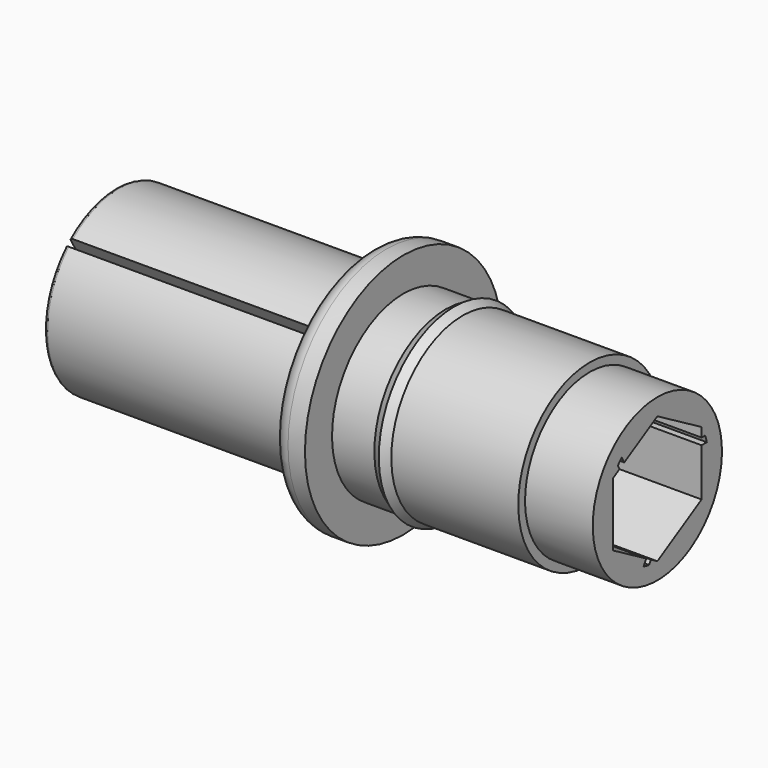
from build123d import *

# Parameters (mm, degrees)
F2_R     = 1
F4_DEPTH = 32
F5_DEPTH = 32
F6_DEPTH = 15
F7_DEPTH = 15
F8_DEPTH = 15
F9_R     = 0.2


with BuildPart() as f1:
    # F0 (on Front) → F1 (revolve)
    with BuildSketch(Plane.XZ):
        Polygon((-9.0454753935, 5.269), (-9.0454753935, 3.769), (22.9545246065, 3.769), (22.9545246065, 4.769), (18.9545246065, 4.769), (18.9545246065, 5.269), (11.4545246065, 5.269), (10.9545246065, 5.569), (10.4545246065, 5.269), (7.9545246065, 5.269), (7.9545246065, 7.269), (5.9545246065, 7.269), (5.9545246065, 5.269), align=None)
    revolve(axis=Axis((2.1683473801, 0, 0), (1, 0, 0)))

    # F2
    f2_edges = [f1.edges().sort_by_distance(p)[0] for p in [
        (5.954525, 0, -7.269),
    ]]
    fillet(f2_edges, radius=F2_R)

    # F3 (on face) → F4 (join)
    with BuildSketch(Plane(origin=(-9.0454753935, 0, 0), x_dir=(0, -1, 0), z_dir=(-1, 0, 0))):
        with BuildLine():
            ThreePointArc((3.769, 0), (3.6405744393, 0.975488981), (3.2640497469, 1.8845))
            Line((3.2640497469, 1.8845), (3.2640497469, -1.8845))
            ThreePointArc((3.2640497469, -1.8845), (3.6405744393, -0.975488981), (3.769, 0))
        make_face()
    extrude(amount=-F4_DEPTH)

    # F3 (on face) → F5 (join)
    with BuildSketch(Plane(origin=(-9.0454753935, 0, 0), x_dir=(0, -1, 0), z_dir=(-1, 0, 0))):
        with BuildLine():
            ThreePointArc((3.769, 0), (3.6405744393, 0.975488981), (3.2640497469, 1.8845))
            Line((3.2640497469, 1.8845), (3.2640497469, -1.8845))
            ThreePointArc((3.2640497469, -1.8845), (3.6405744393, -0.975488981), (3.769, 0))
        make_face()
        with BuildLine():
            Line((2.7877357748, 2.1595), (3.2640497469, 1.8845))
            ThreePointArc((3.2640497469, 1.8845), (3.1012168176, 2.1419185909), (2.9181290377, 2.3853477564))
            Line((2.9181290377, 2.3853477564), (2.7877357748, 2.1595))
        make_face()
        with BuildLine():
            ThreePointArc((1.0163546733, -3.6293779327), (2.3111934688, -2.9772043514), (3.2640497469, -1.8845))
            Line((3.2640497469, -1.8845), (0.8227241336, -3.294))
            Line((0.8227241336, -3.294), (1.0163546733, -3.6293779327))
        make_face()
        with BuildLine():
            Line((0, 3.769), (2.4413256133, 2.3595))
            Line((2.4413256133, 2.3595), (2.634956153, 2.6948779327))
            ThreePointArc((2.634956153, 2.6948779327), (1.4227378662, 3.4901544327), (0, 3.769))
        make_face()
        with BuildLine():
            Line((0.606707235, -3.7198477564), (0.4763139721, -3.494))
            Line((0.4763139721, -3.494), (0, -3.769))
            ThreePointArc((0, -3.769), (0.3043475037, -3.7566918422), (0.606707235, -3.7198477564))
        make_face()
        with BuildLine():
            Line((-3.2640497469, 1.8845), (0, 3.769))
            ThreePointArc((0, 3.769), (-1.8845, 3.2640497469), (-3.2640497469, 1.8845))
        make_face()
        with BuildLine():
            ThreePointArc((-3.2640497469, -1.8845), (-1.8845, -3.2640497469), (0, -3.769))
            Line((0, -3.769), (-3.2640497469, -1.8845))
        make_face()
        with BuildLine():
            Line((-3.2640497469, 1.3345), (-3.2640497469, 1.8845))
            ThreePointArc((-3.2640497469, 1.8845), (-3.4055643214, 1.6147732513), (-3.5248362728, 1.3345))
            Line((-3.5248362728, 1.3345), (-3.2640497469, 1.3345))
        make_face()
        with BuildLine():
            ThreePointArc((-3.6513108263, 0.9345), (-3.7339313349, -0.5129500813), (-3.2640497469, -1.8845))
            Line((-3.2640497469, -1.8845), (-3.2640497469, 0.9345))
            Line((-3.2640497469, 0.9345), (-3.6513108263, 0.9345))
        make_face()
    extrude(amount=-F5_DEPTH)

    # F3 (on face) → F6 (cut)
    with BuildSketch(Plane(origin=(-9.0454753935, 0, 0), x_dir=(0, -1, 0), z_dir=(-1, 0, 0))):
        with BuildLine():
            ThreePointArc((2.634956153, 2.6948779327), (2.78085257, 2.5440558138), (2.9181290377, 2.3853477564))
            Line((2.9181290377, 2.3853477564), (3.704312025, 3.7470566344))
            ThreePointArc((3.704312025, 3.7470566344), (3.5558605867, 3.8882150774), (3.402034372, 4.0234963814))
            Line((3.402034372, 4.0234963814), (2.634956153, 2.6948779327))
        make_face()
    extrude(amount=-F6_DEPTH, mode=Mode.SUBTRACT)

    # F3 (on face) → F7 (cut)
    with BuildSketch(Plane(origin=(-9.0454753935, 0, 0), x_dir=(0, -1, 0), z_dir=(-1, 0, 0))):
        with BuildLine():
            Line((1.7834328924, -4.9579963814), (1.0163546733, -3.6293779327))
            ThreePointArc((1.0163546733, -3.6293779327), (0.8127906784, -3.6803168767), (0.606707235, -3.7198477564))
            Line((0.606707235, -3.7198477564), (1.3928902223, -5.0815566344))
            ThreePointArc((1.3928902223, -5.0815566344), (1.589362739, -5.0235731391), (1.7834328924, -4.9579963814))
        make_face()
    extrude(amount=-F7_DEPTH, mode=Mode.SUBTRACT)

    # F3 (on face) → F8 (cut)
    with BuildSketch(Plane(origin=(-9.0454753935, 0, 0), x_dir=(0, -1, 0), z_dir=(-1, 0, 0))):
        with BuildLine():
            Line((-3.5248362728, 1.3345), (-5.0972022473, 1.3345))
            ThreePointArc((-5.0972022473, 1.3345), (-5.1452233257, 1.1353580617), (-5.1854672644, 0.9345))
            Line((-5.1854672644, 0.9345), (-3.6513108263, 0.9345))
            ThreePointArc((-3.6513108263, 0.9345), (-3.5936432484, 1.1362610629), (-3.5248362728, 1.3345))
        make_face()
    extrude(amount=-F8_DEPTH, mode=Mode.SUBTRACT)

    # F9
    f9_edges = [f1.edges().sort_by_distance(p)[0] for p in [
        (-9.045475, 1.589363, 5.023573),
        (-9.045475, -5.145223, -1.135358),
        (-9.045475, 3.555861, -3.888215),
        (-9.045475, 3.26405, -0.475),
        (-9.045475, 1.632025, -2.82675),
        (-9.045475, -0.238157, -3.6315),
        (-9.045475, -3.26405, 0),
        (-9.045475, -3.025893, 2.022),
        (-9.045475, 1.632025, 2.82675),
        (-9.045475, -1.220663, 3.06425),
        (-9.045475, -2.043387, -2.58925),
        (-9.045475, 3.26405, 1.6095),
    ]]
    fillet(f9_edges, radius=F9_R)


solid = f1.part
